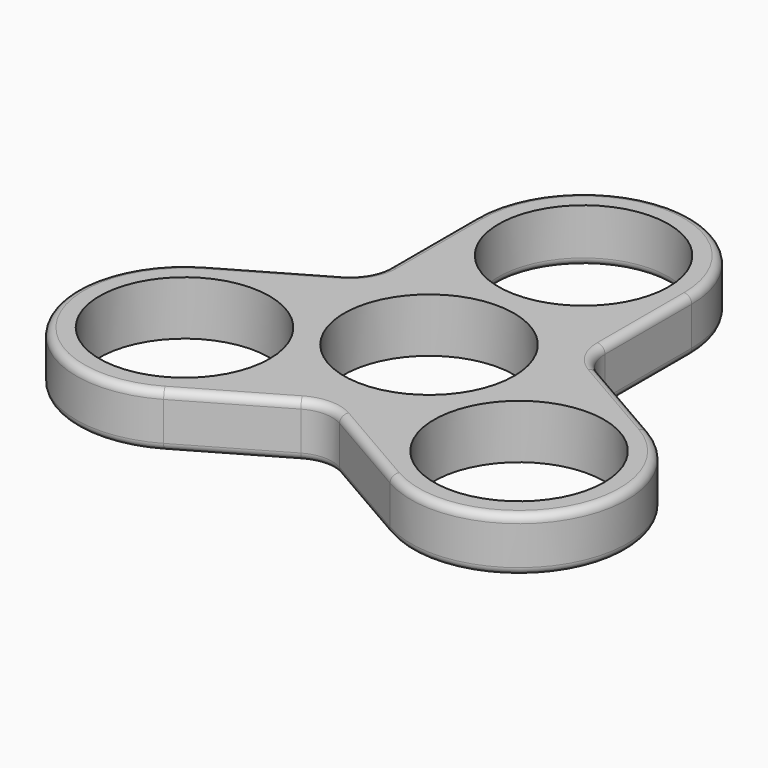
from build123d import *

# Parameters (mm, degrees)
F0_R     = 11
F1_DEPTH = 3.5
F2_R     = 1
F3_R     = 1


# Not quite as in the source:
# - a feature names something its author has since deleted; it is built from what else it names


with BuildPart() as f1:
    # F0 (on Top) → F1 (new body, symmetric)
    with BuildSketch(Plane.XY):
        with BuildLine():
            ThreePointArc((-28.6506350946, -0.375644347), (-33.7749907476, -19.5), (-14.6506350946, -24.624355653))
            Line((-14.6506350946, -24.624355653), (-2.5, -17.6091832103))
            ThreePointArc((-2.5, -17.6091832103), (0, -16.9393102292), (2.5, -17.6091832103))
            Line((2.5, -17.6091832103), (14.6506350946, -24.624355653))
            ThreePointArc((14.6506350946, -24.624355653), (33.7749907476, -19.5), (28.6506350946, -0.375644347))
            Line((28.6506350946, -0.375644347), (16.5, 6.6395280957))
            ThreePointArc((16.5, 6.6395280957), (14.6698729811, 8.4696551146), (14, 10.9696551146))
            Line((14, 10.9696551146), (14, 25))
            ThreePointArc((14, 25), (0, 39), (-14, 25))
            Line((-14, 25), (-14, 10.9696551146))
            ThreePointArc((-14, 10.9696551146), (-14.6698729811, 8.4696551146), (-16.5, 6.6395280957))
            Line((-16.5, 6.6395280957), (-28.6506350946, -0.375644347))
        make_face()
        with Locations((-21.6506350946, -12.5)):
            Circle(F0_R, mode=Mode.SUBTRACT)
        with Locations((21.6506350946, -12.5)):
            Circle(F0_R, mode=Mode.SUBTRACT)
        Circle(F0_R, mode=Mode.SUBTRACT)
        with Locations((0, 25)):
            Circle(F0_R, mode=Mode.SUBTRACT)
    extrude(amount=F1_DEPTH, both=True)

    # F2
    f2_edges = [f1.edges().sort_by_distance(p)[0] for p in [
        (-8.575318, -21.116769, 3.5),
        (-33.774991, -19.5, 3.5),
        (-22.575318, 3.131942, 3.5),
    ]]
    fillet(f2_edges, radius=F2_R)

    # F3
    f3_edges = [f1.edges().sort_by_distance(p)[0] for p in [
        (-8.575318, -21.116769, -3.5),
        (-33.774991, -19.5, -3.5),
        (-22.575318, 3.131942, -3.5),
        (-11, 25, -3.5),
    ]]
    fillet(f3_edges, radius=F3_R)


solid = f1.part
